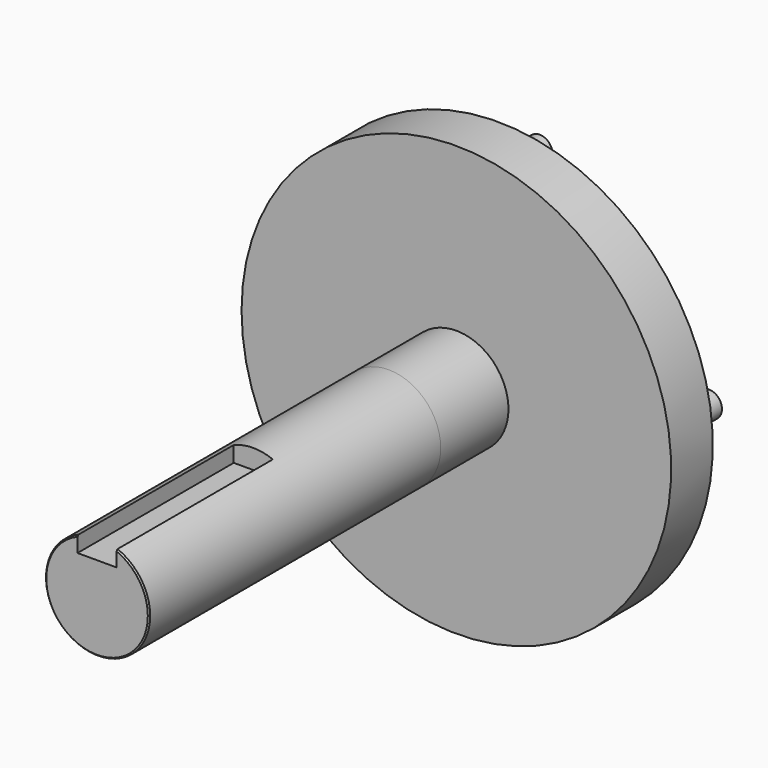
from build123d import *

# Parameters (mm, degrees)
F0_R      = 4
F1_DEPTH  = 28
F2_SIZE   = 0.1
F3_R      = 4
F4_DEPTH  = 6.5
F5_R      = 16.5
F6_DEPTH  = 4
F7_R      = 1
F8_DEPTH  = 4
F9_W      = 3
F9_H      = 1.5
F10_DEPTH = 15


with BuildPart() as f1:
    # F0 (on Front) → F1 (new body)
    with BuildSketch(Plane.XZ):
        Circle(F0_R)
    extrude(amount=-F1_DEPTH)

    # F2
    f2_edges = [f1.edges().sort_by_distance(p)[0] for p in [
        (-4, 0, 0),
    ]]
    chamfer(f2_edges, length=F2_SIZE)

    # F3 (on face) → F4 (join)
    with BuildSketch(Plane(origin=(0, 28, 0), x_dir=(-1, 0, 0), z_dir=(0, 1, 0))):
        Circle(F3_R)
    extrude(amount=F4_DEPTH)

    # F5 (on face) → F6 (join)
    with BuildSketch(Plane(origin=(0, 34.5, 0), x_dir=(-1, 0, 0), z_dir=(0, 1, 0))):
        Circle(F5_R)
    extrude(amount=F6_DEPTH)

    # F7 (on face) → F8 (join)
    with BuildSketch(Plane(origin=(0, 38.5, 0), x_dir=(-1, 0, 0), z_dir=(0, 1, 0))):
        with Locations((0, 13)):
            Circle(F7_R)
        with Locations((-13, 0)):
            Circle(F7_R)
        with Locations((0, -13)):
            Circle(F7_R)
        with Locations((13, 0)):
            Circle(F7_R)
    extrude(amount=F8_DEPTH)

    # F9 (on face) → F10 (cut)
    with BuildSketch(Plane.XZ):
        with Locations((0, 3.25)):
            Rectangle(F9_W, F9_H)
    extrude(amount=-F10_DEPTH, mode=Mode.SUBTRACT)


solid = f1.part
